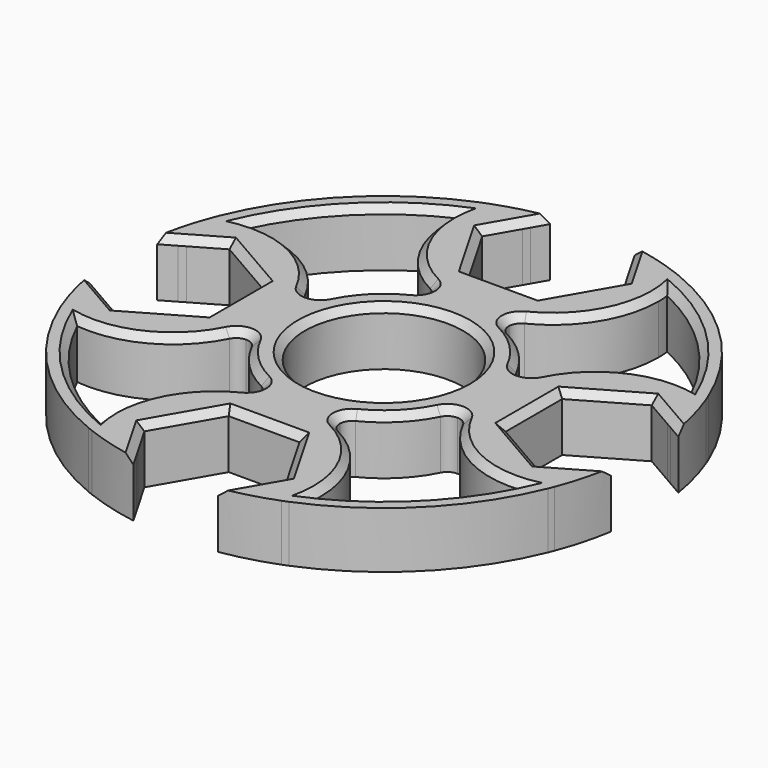
from build123d import *

# Parameters (mm, degrees)
F0_R          = 11.25
F1_DEPTH      = 8
F2_T6_DEPTH   = 13.2460185776
F2_T10_DEPTH  = 15.1933659759
F2_T15_DEPTH  = 15.1933659759
F2_T20_DEPTH  = 15.1933659759
F2_T25_DEPTH  = 13.2460185776
F2_T29_DEPTH  = 15.1933659759
F2_T34_DEPTH  = 13.2460185776
F2_T38_DEPTH  = 15.1933659759
F2_T43_DEPTH  = 15.1933659759
F2_T48_DEPTH  = 13.2460185776
F2_T52_ANGLE  = 79.6397986482
F2_S53_R      = 35
F2_T54_DEPTH  = 11
F2_T57_ANGLE  = 79.6397986482
F2_S58_R      = 35
F2_T59_DEPTH  = 11
F2_T62_ANGLE  = 48.0029281472
F2_S63_R      = 15
F2_T64_DEPTH  = 16
F2_S65_R      = 15
F2_T66_DEPTH  = 16
F2_T69_ANGLE  = 48.0029281472
F2_S70_R      = 15
F2_T71_DEPTH  = 16
F2_S72_R      = 15
F2_T73_DEPTH  = 16
F2_T76_DEPTH  = 13.2460185776
F2_T80_DEPTH  = 15.1933659759
F2_T85_DEPTH  = 15.1933659759
F2_T90_DEPTH  = 15.1933659759
F2_T95_DEPTH  = 13.2460185776
F2_T99_ANGLE  = 79.6397986482
F2_S100_R     = 35
F2_T101_DEPTH = 11
F2_T104_ANGLE = 48.0029281472
F2_S105_R     = 15
F2_T106_DEPTH = 16
F2_S107_R     = 15
F2_T108_DEPTH = 16
F2_T111_DEPTH = 13.2460185776
F2_T115_DEPTH = 15.1933659759
F2_T120_DEPTH = 15.1933659759
F2_T125_DEPTH = 15.1933659759
F2_T130_DEPTH = 13.2460185776
F2_T134_ANGLE = 79.6397986482
F2_S135_R     = 35
F2_T136_DEPTH = 11
F2_T139_ANGLE = 48.0029281472
F2_S140_R     = 15
F2_T141_DEPTH = 16
F2_S142_R     = 15
F2_T143_DEPTH = 16
F2_T146_ANGLE = 79.6397986482
F2_S147_R     = 35
F2_T148_DEPTH = 11
F2_T151_ANGLE = 126.8698976458
F2_T154_ANGLE = 36.8698976458
F2_T157_ANGLE = 126.8698976458
F2_T160_ANGLE = 126.8698976458
F2_T163_ANGLE = 36.8698976458
F2_T166_ANGLE = 126.8698976458
F2_T169_ANGLE = 79.6397986482
F2_S170_R     = 35
F2_T171_DEPTH = 11
F2_T174_ANGLE = 36.8698976458
F2_T177_ANGLE = 126.8698976458
F2_T180_ANGLE = 79.6397986482
F2_S181_R     = 35
F2_T182_DEPTH = 11
F2_T185_ANGLE = 126.8698976458
F2_T188_ANGLE = 36.8698976458
F2_T191_ANGLE = 126.8698976458
F2_T194_ANGLE = 79.6397986482
F2_S195_R     = 35
F2_T196_DEPTH = 11
F2_T199_ANGLE = 126.8698976458
F2_T203_DEPTH = 15.1933659759
F2_T207_DEPTH = 13.2460185776
F2_T213_DEPTH = 15.1933659759
F2_T217_DEPTH = 15.1933659759
F2_T223_DEPTH = 15.1933659759
F2_T227_DEPTH = 15.1933659759
F2_T233_DEPTH = 13.2460185776
F2_T237_DEPTH = 15.1933659759
F2_T243_DEPTH = 15.1933659759
F2_T247_DEPTH = 15.1933659759
F2_T253_DEPTH = 15.1933659759
F2_T257_DEPTH = 13.2460185776
F2_T263_DEPTH = 15.1933659759
F2_T267_DEPTH = 15.1933659759
F2_T273_DEPTH = 13.2460185776
F2_T277_DEPTH = 15.1933659759
F2_T283_ANGLE = 79.6397986482
F2_S284_R     = 35
F2_T285_DEPTH = 11
F2_T288_ANGLE = 48.0029281472
F2_S289_R     = 15
F2_T290_DEPTH = 16
F2_T295_ANGLE = 79.6397986482
F2_S296_R     = 35
F2_T297_DEPTH = 11
F2_T300_ANGLE = 48.0029281472
F2_S301_R     = 15
F2_T302_DEPTH = 16
F2_T307_ANGLE = 48.0029281472
F2_S308_R     = 15
F2_T309_DEPTH = 16
F2_T312_ANGLE = 79.6397986482
F2_S313_R     = 35
F2_T314_DEPTH = 11
F2_T319_ANGLE = 48.0029281472
F2_S320_R     = 15
F2_T321_DEPTH = 16
F2_T324_ANGLE = 79.6397986482
F2_S325_R     = 35
F2_T326_DEPTH = 11
F2_T331_DEPTH = 15.1933659759
F2_T335_DEPTH = 13.2460185776
F2_T341_DEPTH = 15.1933659759
F2_T345_DEPTH = 15.1933659759
F2_T351_DEPTH = 15.1933659759
F2_T355_DEPTH = 15.1933659759
F2_T361_DEPTH = 13.2460185776
F2_T365_DEPTH = 15.1933659759
F2_T371_ANGLE = 79.6397986482
F2_S372_R     = 35
F2_T373_DEPTH = 11
F2_T376_ANGLE = 48.0029281472
F2_S377_R     = 15
F2_T378_DEPTH = 16
F2_T383_ANGLE = 79.6397986482
F2_S384_R     = 35
F2_T385_DEPTH = 11
F2_T388_ANGLE = 48.0029281472
F2_S389_R     = 15
F2_T390_DEPTH = 16
F2_T395_DEPTH = 15.1933659759
F2_T399_DEPTH = 13.2460185776
F2_T405_DEPTH = 15.1933659759
F2_T409_DEPTH = 15.1933659759
F2_T415_DEPTH = 15.1933659759
F2_T419_DEPTH = 15.1933659759
F2_T425_DEPTH = 15.1933659759
F2_T429_DEPTH = 13.2460185776
F2_T435_ANGLE = 79.6397986482
F2_S436_R     = 35
F2_T437_DEPTH = 11
F2_T440_ANGLE = 48.0029281472
F2_S441_R     = 15
F2_T442_DEPTH = 16
F2_T447_ANGLE = 48.0029281472
F2_S448_R     = 15
F2_T449_DEPTH = 16
F2_T452_ANGLE = 79.6397986482
F2_S453_R     = 35
F2_T454_DEPTH = 11


# Not quite as in the source:
# - a fillet or chamfer that OpenCascade refuses, or shapes differently, is made with other operations: its cross-section is extruded or revolved along the edge and cut away or added


with BuildPart() as f1:
    # F0 (on Top) → F1 (new body)
    with BuildSketch(Plane.XY):
        with BuildLine():
            ThreePointArc((-16.583592135, 6.7082039325), (-22.8362258472, 13.1787837029), (-31.6666666667, 14.90711985))
            ThreePointArc((-31.6666666667, 14.90711985), (-33.1092804377, 11.3479314811), (-34.1532596523, 7.6521144217))
            Line((-34.1532596523, 7.6521144217), (-30, 10.05))
            Line((-30, 10.05), (-21.296444692, 5.025))
            Line((-21.296444692, 5.025), (-21.296444692, 0))
            Line((-21.296444692, 0), (-15, 0))
            ThreePointArc((-15, 0), (-15.401265158, 3.4462938082), (-16.583592135, 6.7082039325))
        make_face()
        with BuildLine():
            ThreePointArc((-34.1532596523, -7.6521144217), (-33.1092804377, -11.3479314811), (-31.6666666667, -14.90711985))
            ThreePointArc((-31.6666666667, -14.90711985), (-22.8362258472, -13.1787837029), (-16.583592135, -6.7082039325))
            ThreePointArc((-16.583592135, -6.7082039325), (-15.401265158, -3.4462938082), (-15, 0))
            Line((-15, 0), (-21.296444692, 0))
            Line((-21.296444692, 0), (-21.296444692, -5.025))
            Line((-21.296444692, -5.025), (-30, -10.05))
            Line((-30, -10.05), (-34.1532596523, -7.6521144217))
        make_face()
        with BuildLine():
            ThreePointArc((-34.6875, -14.248766394), (-33.1940907666, -14.6559811741), (-31.6666666667, -14.90711985))
            ThreePointArc((-31.6666666667, -14.90711985), (-33.1092804377, -11.3479314811), (-34.1532596523, -7.6521144217))
            Line((-34.1532596523, -7.6521144217), (-35, -7.1632486541))
            Line((-35, -7.1632486541), (-35, -13.4629120178))
            ThreePointArc((-35, -13.4629120178), (-34.8459654169, -13.8567201806), (-34.6875, -14.248766394))
        make_face()
        with BuildLine():
            ThreePointArc((-37.0171029911, -5.9986736992), (-36.2014432616, -9.7829190825), (-35, -13.4629120178))
            Line((-35, -13.4629120178), (-35, -7.1632486541))
            Line((-35, -7.1632486541), (-37.0171029911, -5.9986736992))
        make_face()
        with BuildLine():
            Line((-35, 7.1632486541), (-35, 13.4629120178))
            ThreePointArc((-35, 13.4629120178), (-36.2014432616, 9.7829190825), (-37.0171029911, 5.9986736992))
            Line((-37.0171029911, 5.9986736992), (-35, 7.1632486541))
        make_face()
        with BuildLine():
            ThreePointArc((-34.1532596523, 7.6521144217), (-33.1092804377, 11.3479314811), (-31.6666666667, 14.90711985))
            ThreePointArc((-31.6666666667, 14.90711985), (-33.1940907666, 14.6559811741), (-34.6875, 14.248766394))
            ThreePointArc((-34.6875, 14.248766394), (-34.8459654169, 13.8567201806), (-35, 13.4629120178))
            Line((-35, 13.4629120178), (-35, 7.1632486541))
            Line((-35, 7.1632486541), (-34.1532596523, 7.6521144217))
        make_face()
        with BuildLine():
            ThreePointArc((-31.6666666667, 14.90711985), (-24.7487373415, 24.7487373415), (-14.90711985, 31.6666666667))
            ThreePointArc((-14.90711985, 31.6666666667), (-14.6559811741, 33.1940907666), (-14.248766394, 34.6875))
            ThreePointArc((-14.248766394, 34.6875), (-26.5165042945, 26.5165042945), (-34.6875, 14.248766394))
            ThreePointArc((-34.6875, 14.248766394), (-33.1940907666, 14.6559811741), (-31.6666666667, 14.90711985))
        make_face()
        with BuildLine():
            ThreePointArc((-14.248766394, -34.6875), (-14.6559811741, -33.1940907666), (-14.90711985, -31.6666666667))
            ThreePointArc((-14.90711985, -31.6666666667), (-24.7487373415, -24.7487373415), (-31.6666666667, -14.90711985))
            ThreePointArc((-31.6666666667, -14.90711985), (-33.1940907666, -14.6559811741), (-34.6875, -14.248766394))
            ThreePointArc((-34.6875, -14.248766394), (-26.5165042945, -26.5165042945), (-14.248766394, -34.6875))
        make_face()
        with BuildLine():
            Line((-15, -5.7294901688), (-15, 0))
            ThreePointArc((-15, 0), (-15.401265158, -3.4462938082), (-16.583592135, -6.7082039325))
            ThreePointArc((-16.583592135, -6.7082039325), (-15.9308121026, -5.9939143809), (-15, -5.7294901688))
        make_face()
        with BuildLine():
            ThreePointArc((-15, -5.7294901688), (-14.0691878974, -5.9939143809), (-13.416407865, -6.7082039325))
            ThreePointArc((-13.416407865, -6.7082039325), (-14.598734842, -3.4462938082), (-15, 0))
            Line((-15, 0), (-15, -5.7294901688))
        make_face()
        with BuildLine():
            ThreePointArc((-15, 5.7294901688), (-15.9308121026, 5.9939143809), (-16.583592135, 6.7082039325))
            ThreePointArc((-16.583592135, 6.7082039325), (-15.401265158, 3.4462938082), (-15, 0))
            Line((-15, 0), (-15, 5.7294901688))
        make_face()
        with BuildLine():
            ThreePointArc((-15, 0), (-14.598734842, 3.4462938082), (-13.416407865, 6.7082039325))
            ThreePointArc((-13.416407865, 6.7082039325), (-14.0691878974, 5.9939143809), (-15, 5.7294901688))
            Line((-15, 5.7294901688), (-15, 0))
        make_face()
        with BuildLine():
            ThreePointArc((-14.90711985, -31.6666666667), (-11.3479314811, -33.1092804377), (-7.6521144217, -34.1532596523))
            Line((-7.6521144217, -34.1532596523), (-10.05, -30))
            Line((-10.05, -30), (-5.025, -21.296444692))
            Line((-5.025, -21.296444692), (0, -21.296444692))
            Line((0, -21.296444692), (0, -15))
            ThreePointArc((0, -15), (-3.4462938082, -15.401265158), (-6.7082039325, -16.583592135))
            ThreePointArc((-6.7082039325, -16.583592135), (-13.1787837029, -22.8362258472), (-14.90711985, -31.6666666667))
        make_face()
        with BuildLine():
            Line((-7.1632486541, -35), (-7.6521144217, -34.1532596523))
            ThreePointArc((-7.6521144217, -34.1532596523), (-11.3479314811, -33.1092804377), (-14.90711985, -31.6666666667))
            ThreePointArc((-14.90711985, -31.6666666667), (-14.6559811741, -33.1940907666), (-14.248766394, -34.6875))
            ThreePointArc((-14.248766394, -34.6875), (-13.8567201806, -34.8459654169), (-13.4629120178, -35))
            Line((-13.4629120178, -35), (-7.1632486541, -35))
        make_face()
        with BuildLine():
            Line((-5.9986736992, -37.0171029911), (-7.1632486541, -35))
            Line((-7.1632486541, -35), (-13.4629120178, -35))
            ThreePointArc((-13.4629120178, -35), (-9.7829190825, -36.2014432616), (-5.9986736992, -37.0171029911))
        make_face()
        with BuildLine():
            Line((13.4629120178, -35), (7.1632486541, -35))
            Line((7.1632486541, -35), (5.9986736992, -37.0171029911))
            ThreePointArc((5.9986736992, -37.0171029911), (9.7829190825, -36.2014432616), (13.4629120178, -35))
        make_face()
        with BuildLine():
            ThreePointArc((14.248766394, -34.6875), (14.6559811741, -33.1940907666), (14.90711985, -31.6666666667))
            ThreePointArc((14.90711985, -31.6666666667), (11.3479314811, -33.1092804377), (7.6521144217, -34.1532596523))
            Line((7.6521144217, -34.1532596523), (7.1632486541, -35))
            Line((7.1632486541, -35), (13.4629120178, -35))
            ThreePointArc((13.4629120178, -35), (13.8567201806, -34.8459654169), (14.248766394, -34.6875))
        make_face()
        with BuildLine():
            ThreePointArc((7.6521144217, -34.1532596523), (11.3479314811, -33.1092804377), (14.90711985, -31.6666666667))
            ThreePointArc((14.90711985, -31.6666666667), (14.9767619623, -30.8346263386), (15, -30))
            ThreePointArc((15, -30), (12.7597621253, -22.1140333182), (6.7082039325, -16.583592135))
            ThreePointArc((6.7082039325, -16.583592135), (3.4462938082, -15.401265158), (0, -15))
            Line((0, -15), (0, -21.296444692))
            Line((0, -21.296444692), (5.025, -21.296444692))
            Line((5.025, -21.296444692), (10.05, -30))
            Line((10.05, -30), (7.6521144217, -34.1532596523))
        make_face()
        with BuildLine():
            ThreePointArc((34.6875, -14.248766394), (33.1940907666, -14.6559811741), (31.6666666667, -14.90711985))
            ThreePointArc((31.6666666667, -14.90711985), (24.7487373415, -24.7487373415), (14.90711985, -31.6666666667))
            ThreePointArc((14.90711985, -31.6666666667), (14.6559811741, -33.1940907666), (14.248766394, -34.6875))
            ThreePointArc((14.248766394, -34.6875), (26.5165042945, -26.5165042945), (34.6875, -14.248766394))
        make_face()
        with BuildLine():
            Line((35, -7.1632486541), (34.1532596523, -7.6521144217))
            ThreePointArc((34.1532596523, -7.6521144217), (33.1092804377, -11.3479314811), (31.6666666667, -14.90711985))
            ThreePointArc((31.6666666667, -14.90711985), (33.1940907666, -14.6559811741), (34.6875, -14.248766394))
            ThreePointArc((34.6875, -14.248766394), (34.8459654169, -13.8567201806), (35, -13.4629120178))
            Line((35, -13.4629120178), (35, -7.1632486541))
        make_face()
        with BuildLine():
            Line((37.0171029911, -5.9986736992), (35, -7.1632486541))
            Line((35, -7.1632486541), (35, -13.4629120178))
            ThreePointArc((35, -13.4629120178), (36.2014432616, -9.7829190825), (37.0171029911, -5.9986736992))
        make_face()
        with BuildLine():
            ThreePointArc((31.6666666667, -14.90711985), (33.1092804377, -11.3479314811), (34.1532596523, -7.6521144217))
            Line((34.1532596523, -7.6521144217), (30, -10.05))
            Line((30, -10.05), (21.296444692, -5.025))
            Line((21.296444692, -5.025), (21.296444692, 0))
            Line((21.296444692, 0), (15, 0))
            ThreePointArc((15, 0), (15.401265158, -3.4462938082), (16.583592135, -6.7082039325))
            ThreePointArc((16.583592135, -6.7082039325), (22.8362258472, -13.1787837029), (31.6666666667, -14.90711985))
        make_face()
        with BuildLine():
            Line((30, 10.05), (34.1532596523, 7.6521144217))
            ThreePointArc((34.1532596523, 7.6521144217), (33.1092804377, 11.3479314811), (31.6666666667, 14.90711985))
            ThreePointArc((31.6666666667, 14.90711985), (22.8362258472, 13.1787837029), (16.583592135, 6.7082039325))
            ThreePointArc((16.583592135, 6.7082039325), (15.401265158, 3.4462938082), (15, 0))
            Line((15, 0), (21.296444692, 0))
            Line((21.296444692, 0), (21.296444692, 5.025))
            Line((21.296444692, 5.025), (30, 10.05))
        make_face()
        with BuildLine():
            ThreePointArc((31.6666666667, 14.90711985), (33.1092804377, 11.3479314811), (34.1532596523, 7.6521144217))
            Line((34.1532596523, 7.6521144217), (35, 7.1632486541))
            Line((35, 7.1632486541), (35, 13.4629120178))
            ThreePointArc((35, 13.4629120178), (34.8459654169, 13.8567201806), (34.6875, 14.248766394))
            ThreePointArc((34.6875, 14.248766394), (33.1940907666, 14.6559811741), (31.6666666667, 14.90711985))
        make_face()
        with BuildLine():
            Line((35, 13.4629120178), (35, 7.1632486541))
            Line((35, 7.1632486541), (37.0171029911, 5.9986736992))
            ThreePointArc((37.0171029911, 5.9986736992), (36.2014432616, 9.7829190825), (35, 13.4629120178))
        make_face()
        with BuildLine():
            ThreePointArc((14.90711985, 31.6666666667), (24.7487373415, 24.7487373415), (31.6666666667, 14.90711985))
            ThreePointArc((31.6666666667, 14.90711985), (33.1940907666, 14.6559811741), (34.6875, 14.248766394))
            ThreePointArc((34.6875, 14.248766394), (26.5165042945, 26.5165042945), (14.248766394, 34.6875))
            ThreePointArc((14.248766394, 34.6875), (14.6559811741, 33.1940907666), (14.90711985, 31.6666666667))
        make_face()
        with BuildLine():
            ThreePointArc((7.6521144217, 34.1532596523), (11.3479314811, 33.1092804377), (14.90711985, 31.6666666667))
            ThreePointArc((14.90711985, 31.6666666667), (14.6559811741, 33.1940907666), (14.248766394, 34.6875))
            ThreePointArc((14.248766394, 34.6875), (13.8567201806, 34.8459654169), (13.4629120178, 35))
            Line((13.4629120178, 35), (7.1632486541, 35))
            Line((7.1632486541, 35), (7.6521144217, 34.1532596523))
        make_face()
        with BuildLine():
            Line((5.9986736992, 37.0171029911), (7.1632486541, 35))
            Line((7.1632486541, 35), (13.4629120178, 35))
            ThreePointArc((13.4629120178, 35), (9.7829190825, 36.2014432616), (5.9986736992, 37.0171029911))
        make_face()
        with BuildLine():
            ThreePointArc((15, 30), (14.9767619623, 30.8346263386), (14.90711985, 31.6666666667))
            ThreePointArc((14.90711985, 31.6666666667), (11.3479314811, 33.1092804377), (7.6521144217, 34.1532596523))
            Line((7.6521144217, 34.1532596523), (10.05, 30))
            Line((10.05, 30), (5.025, 21.296444692))
            Line((5.025, 21.296444692), (0, 21.296444692))
            Line((0, 21.296444692), (0, 15))
            ThreePointArc((0, 15), (3.4462938082, 15.401265158), (6.7082039325, 16.583592135))
            ThreePointArc((6.7082039325, 16.583592135), (12.7597621253, 22.1140333182), (15, 30))
        make_face()
        with BuildLine():
            Line((-10.05, 30), (-7.6521144217, 34.1532596523))
            ThreePointArc((-7.6521144217, 34.1532596523), (-11.3479314811, 33.1092804377), (-14.90711985, 31.6666666667))
            ThreePointArc((-14.90711985, 31.6666666667), (-13.1787837029, 22.8362258472), (-6.7082039325, 16.583592135))
            ThreePointArc((-6.7082039325, 16.583592135), (-3.4462938082, 15.401265158), (0, 15))
            Line((0, 15), (0, 21.296444692))
            Line((0, 21.296444692), (-5.025, 21.296444692))
            Line((-5.025, 21.296444692), (-10.05, 30))
        make_face()
        with BuildLine():
            ThreePointArc((-14.90711985, 31.6666666667), (-11.3479314811, 33.1092804377), (-7.6521144217, 34.1532596523))
            Line((-7.6521144217, 34.1532596523), (-7.1632486541, 35))
            Line((-7.1632486541, 35), (-13.4629120178, 35))
            ThreePointArc((-13.4629120178, 35), (-13.8567201806, 34.8459654169), (-14.248766394, 34.6875))
            ThreePointArc((-14.248766394, 34.6875), (-14.6559811741, 33.1940907666), (-14.90711985, 31.6666666667))
        make_face()
        with BuildLine():
            Line((-13.4629120178, 35), (-7.1632486541, 35))
            Line((-7.1632486541, 35), (-5.9986736992, 37.0171029911))
            ThreePointArc((-5.9986736992, 37.0171029911), (-9.7829190825, 36.2014432616), (-13.4629120178, 35))
        make_face()
        with BuildLine():
            ThreePointArc((-6.7082039325, 13.416407865), (-3.4462938082, 14.598734842), (0, 15))
            Line((0, 15), (-5.7294901688, 15))
            ThreePointArc((-5.7294901688, 15), (-5.9939143809, 14.0691878974), (-6.7082039325, 13.416407865))
        make_face()
        with BuildLine():
            Line((-5.7294901688, 15), (0, 15))
            ThreePointArc((0, 15), (-3.4462938082, 15.401265158), (-6.7082039325, 16.583592135))
            ThreePointArc((-6.7082039325, 16.583592135), (-5.9939143809, 15.9308121026), (-5.7294901688, 15))
        make_face()
        with BuildLine():
            ThreePointArc((5.7294901688, 15), (5.9939143809, 15.9308121026), (6.7082039325, 16.583592135))
            ThreePointArc((6.7082039325, 16.583592135), (3.4462938082, 15.401265158), (0, 15))
            Line((0, 15), (5.7294901688, 15))
        make_face()
        with BuildLine():
            ThreePointArc((0, 15), (3.4462938082, 14.598734842), (6.7082039325, 13.416407865))
            ThreePointArc((6.7082039325, 13.416407865), (5.9939143809, 14.0691878974), (5.7294901688, 15))
            Line((5.7294901688, 15), (0, 15))
        make_face()
        with BuildLine():
            ThreePointArc((15, 0), (15.401265158, 3.4462938082), (16.583592135, 6.7082039325))
            ThreePointArc((16.583592135, 6.7082039325), (15.9308121026, 5.9939143809), (15, 5.7294901688))
            Line((15, 5.7294901688), (15, 0))
        make_face()
        with BuildLine():
            ThreePointArc((13.416407865, 6.7082039325), (14.598734842, 3.4462938082), (15, 0))
            Line((15, 0), (15, 5.7294901688))
            ThreePointArc((15, 5.7294901688), (14.0691878974, 5.9939143809), (13.416407865, 6.7082039325))
        make_face()
        with BuildLine():
            Line((15, -5.7294901688), (15, 0))
            ThreePointArc((15, 0), (14.598734842, -3.4462938082), (13.416407865, -6.7082039325))
            ThreePointArc((13.416407865, -6.7082039325), (14.0691878974, -5.9939143809), (15, -5.7294901688))
        make_face()
        with BuildLine():
            ThreePointArc((5.7294901688, -15), (5.9939143809, -14.0691878974), (6.7082039325, -13.416407865))
            ThreePointArc((6.7082039325, -13.416407865), (3.4462938082, -14.598734842), (0, -15))
            Line((0, -15), (5.7294901688, -15))
        make_face()
        with BuildLine():
            ThreePointArc((0, -15), (3.4462938082, -15.401265158), (6.7082039325, -16.583592135))
            ThreePointArc((6.7082039325, -16.583592135), (5.9939143809, -15.9308121026), (5.7294901688, -15))
            Line((5.7294901688, -15), (0, -15))
        make_face()
        with BuildLine():
            ThreePointArc((15, -5.7294901688), (15.9308121026, -5.9939143809), (16.583592135, -6.7082039325))
            ThreePointArc((16.583592135, -6.7082039325), (15.401265158, -3.4462938082), (15, 0))
            Line((15, 0), (15, -5.7294901688))
        make_face()
        with BuildLine():
            ThreePointArc((13.416407865, -6.7082039325), (14.598734842, -3.4462938082), (15, 0))
            ThreePointArc((15, 0), (14.598734842, 3.4462938082), (13.416407865, 6.7082039325))
            ThreePointArc((13.416407865, 6.7082039325), (10.6066017178, 10.6066017178), (6.7082039325, 13.416407865))
            ThreePointArc((6.7082039325, 13.416407865), (3.4462938082, 14.598734842), (0, 15))
            ThreePointArc((0, 15), (-3.4462938082, 14.598734842), (-6.7082039325, 13.416407865))
            ThreePointArc((-6.7082039325, 13.416407865), (-10.6066017178, 10.6066017178), (-13.416407865, 6.7082039325))
            ThreePointArc((-13.416407865, 6.7082039325), (-14.598734842, 3.4462938082), (-15, 0))
            ThreePointArc((-15, 0), (-14.598734842, -3.4462938082), (-13.416407865, -6.7082039325))
            ThreePointArc((-13.416407865, -6.7082039325), (-10.6066017178, -10.6066017178), (-6.7082039325, -13.416407865))
            ThreePointArc((-6.7082039325, -13.416407865), (-3.4462938082, -14.598734842), (0, -15))
            ThreePointArc((0, -15), (3.4462938082, -14.598734842), (6.7082039325, -13.416407865))
            ThreePointArc((6.7082039325, -13.416407865), (10.6066017178, -10.6066017178), (13.416407865, -6.7082039325))
        make_face()
        Circle(F0_R, mode=Mode.SUBTRACT)
        with BuildLine():
            ThreePointArc((-6.7082039325, -16.583592135), (-3.4462938082, -15.401265158), (0, -15))
            Line((0, -15), (-5.7294901688, -15))
            ThreePointArc((-5.7294901688, -15), (-5.9939143809, -15.9308121026), (-6.7082039325, -16.583592135))
        make_face()
        with BuildLine():
            Line((-5.7294901688, -15), (0, -15))
            ThreePointArc((0, -15), (-3.4462938082, -14.598734842), (-6.7082039325, -13.416407865))
            ThreePointArc((-6.7082039325, -13.416407865), (-5.9939143809, -14.0691878974), (-5.7294901688, -15))
        make_face()
    extrude(amount=F1_DEPTH)

    # F2: chamfer of 1 on 45 edges, made by hand


with BuildPart() as f2_tool1:
    # F2_s2 → F2_t3 (revolve)
    with BuildSketch(Plane.XZ):
        Polygon((11.25, 7), (12.25, 8), (11.25, 8), align=None)
    revolve(axis=Axis((0, 0, 8), (0, 0, 1)))


with BuildPart() as f2_tool4:
    # F2_s5 → F2_t6 (new body)
    with BuildSketch(Plane(origin=(9.1920395628, 15.9210795479, 0), x_dir=(0, 0, 1), z_dir=(0.5, 0.8660254038, 0))):
        Polygon((7, -23.703555308), (8, -24.703555308), (8, -23.703555308), align=None)
    extrude(amount=F2_T6_DEPTH)

    split(bisect_by=Plane(origin=(5.4528810568, 3.148222346, 0), x_dir=(0, 0, 1), z_dir=(0.8660254038, 0.5, 0)), keep=Keep.TOP)


with BuildPart() as f2_tool8:
    # F2_s9 → F2_t10 (new body)
    with BuildSketch(Plane(origin=(-9.1920395628, 15.9210795479, 0), x_dir=(0, 0, 1), z_dir=(-0.5, 0.8660254038, 0))):
        Polygon((7, 6.296444692), (8, 5.296444692), (8, 6.296444692), align=None)
    extrude(amount=F2_T10_DEPTH)

    split(bisect_by=Plane.XZ.offset(-21.296444692), keep=Keep.BOTTOM)

    split(bisect_by=Plane(origin=(-20.5278810568, 11.851777654, 0), x_dir=(0, 0, 1), z_dir=(0.8660254038, -0.5, 0)), keep=Keep.TOP)


with BuildPart() as f2_tool13:
    # F2_s14 → F2_t15 (new body)
    with BuildSketch(Plane.YZ.offset(7.596682988)):
        Polygon((21.296444692, 7), (20.296444692, 8), (21.296444692, 8), align=None)
    extrude(amount=-F2_T15_DEPTH)

    split(bisect_by=Plane(origin=(-5.4528810568, 3.148222346, 0), x_dir=(0, 0, 1), z_dir=(-0.8660254038, 0.5, 0)), keep=Keep.TOP)

    split(bisect_by=Plane(origin=(5.4528810568, 3.148222346, 0), x_dir=(0, 0, 1), z_dir=(0.8660254038, 0.5, 0)), keep=Keep.TOP)


with BuildPart() as f2_tool18:
    # F2_s19 → F2_t20 (new body)
    with BuildSketch(Plane(origin=(16.7887225507, 29.0789204521, 0), x_dir=(0, 0, 1), z_dir=(-0.5, -0.8660254038, 0))):
        Polygon((7, 6.296444692), (8, 5.296444692), (8, 6.296444692), align=None)
    extrude(amount=F2_T20_DEPTH)

    split(bisect_by=Plane(origin=(20.5278810568, 11.851777654, 0), x_dir=(0, 0, 1), z_dir=(-0.8660254038, -0.5, 0)), keep=Keep.TOP)

    split(bisect_by=Plane.XZ.offset(-21.296444692), keep=Keep.BOTTOM)


with BuildPart() as f2_tool23:
    # F2_s24 → F2_t25 (new body)
    with BuildSketch(Plane(origin=(-15.8150488516, 27.3924681351, 0), x_dir=(0, 0, 1), z_dir=(0.5, -0.8660254038, 0))):
        Polygon((7, -23.703555308), (8, -24.703555308), (8, -23.703555308), align=None)
    extrude(amount=F2_T25_DEPTH)

    split(bisect_by=Plane(origin=(-5.4528810568, 3.148222346, 0), x_dir=(0, 0, 1), z_dir=(-0.8660254038, 0.5, 0)), keep=Keep.TOP)


with BuildPart() as f2_tool27:
    # F2_s28 → F2_t29 (new body)
    with BuildSketch(Plane(origin=(15.9210795479, 9.1920395628, 0), x_dir=(0, 0, 1), z_dir=(0.8660254038, 0.5, 0))):
        Polygon((7, 6.296444692), (8, 5.296444692), (8, 6.296444692), align=None)
    extrude(amount=F2_T29_DEPTH)

    split(bisect_by=Plane.YZ.offset(21.296444692), keep=Keep.TOP)

    split(bisect_by=Plane(origin=(11.851777654, 20.5278810568, 0), x_dir=(0, 0, 1), z_dir=(-0.5, -0.8660254038, 0)), keep=Keep.TOP)


with BuildPart() as f2_tool32:
    # F2_s33 → F2_t34 (new body)
    with BuildSketch(Plane(origin=(15.9210795479, -9.1920395628, 0), x_dir=(0, 0, 1), z_dir=(0.8660254038, -0.5, 0))):
        Polygon((7, -23.703555308), (8, -24.703555308), (8, -23.703555308), align=None)
    extrude(amount=F2_T34_DEPTH)

    split(bisect_by=Plane(origin=(3.148222346, -5.4528810568, 0), x_dir=(0, 0, 1), z_dir=(0.5, -0.8660254038, 0)), keep=Keep.TOP)


with BuildPart() as f2_tool36:
    # F2_s37 → F2_t38 (new body)
    with BuildSketch(Plane.XZ.offset(7.596682988)):
        Polygon((21.296444692, 7), (20.296444692, 8), (21.296444692, 8), align=None)
    extrude(amount=-F2_T38_DEPTH)

    split(bisect_by=Plane(origin=(3.148222346, 5.4528810568, 0), x_dir=(0, 0, 1), z_dir=(0.5, 0.8660254038, 0)), keep=Keep.TOP)

    split(bisect_by=Plane(origin=(3.148222346, -5.4528810568, 0), x_dir=(0, 0, 1), z_dir=(0.5, -0.8660254038, 0)), keep=Keep.TOP)


with BuildPart() as f2_tool41:
    # F2_s42 → F2_t43 (new body)
    with BuildSketch(Plane(origin=(29.0789204521, -16.7887225507, 0), x_dir=(0, 0, 1), z_dir=(-0.8660254038, 0.5, 0))):
        Polygon((7, 6.296444692), (8, 5.296444692), (8, 6.296444692), align=None)
    extrude(amount=F2_T43_DEPTH)

    split(bisect_by=Plane(origin=(11.851777654, -20.5278810568, 0), x_dir=(0, 0, 1), z_dir=(-0.5, 0.8660254038, 0)), keep=Keep.TOP)

    split(bisect_by=Plane.YZ.offset(21.296444692), keep=Keep.TOP)


with BuildPart() as f2_tool46:
    # F2_s47 → F2_t48 (new body)
    with BuildSketch(Plane(origin=(27.3924681351, 15.8150488516, 0), x_dir=(0, 0, 1), z_dir=(-0.8660254038, -0.5, 0))):
        Polygon((7, -23.703555308), (8, -24.703555308), (8, -23.703555308), align=None)
    extrude(amount=F2_T48_DEPTH)

    split(bisect_by=Plane(origin=(3.148222346, 5.4528810568, 0), x_dir=(0, 0, 1), z_dir=(0.5, 0.8660254038, 0)), keep=Keep.TOP)


with BuildPart() as f2_tool50:
    # F2_s51 → F2_t52 (revolve)
    with BuildSketch(Plane(origin=(6, -12, 0), x_dir=(0, 0, 1), z_dir=(-0.4472135955, 0.894427191, 0))):
        Polygon((7, 11.83281573), (8, 12.83281573), (8, 11.83281573), align=None)
    revolve(axis=Axis((30, 0, 8), (0, 0, 1)), revolution_arc=F2_T52_ANGLE)

    # F2_s53 → F2_t54 (intersect, symmetric)
    with BuildSketch(Plane.XY.offset(7.5)):
        Circle(F2_S53_R)
    extrude(amount=F2_T54_DEPTH, both=True, mode=Mode.INTERSECT)


with BuildPart() as f2_tool55:
    # F2_s56 → F2_t57 (revolve)
    with BuildSketch(Plane(origin=(12, 6, 0), x_dir=(0, 0, 1), z_dir=(-0.894427191, -0.4472135955, 0))):
        Polygon((7, 11.83281573), (8, 12.83281573), (8, 11.83281573), align=None)
    revolve(axis=Axis((0, 30, 8), (0, 0, 1)), revolution_arc=F2_T57_ANGLE)

    # F2_s58 → F2_t59 (intersect, symmetric)
    with BuildSketch(Plane.XY.offset(7.5)):
        Circle(F2_S58_R)
    extrude(amount=F2_T59_DEPTH, both=True, mode=Mode.INTERSECT)


with BuildPart() as f2_tool60:
    # F2_s61 → F2_t62 (revolve)
    with BuildSketch(Plane(origin=(0, 0, 0), x_dir=(0, 0, 1), z_dir=(0.3583440937, 0.9335895835, 0))):
        Polygon((7, 35), (8, 36), (8, 35), align=None)
    revolve(axis=Axis((0, 0, 8), (0, 0, -1)), revolution_arc=F2_T62_ANGLE)

    # F2_s63 → F2_t64 (cut, symmetric)
    with BuildSketch(Plane.XY.offset(7.5)):
        with Locations((30, 0)):
            Circle(F2_S63_R)
    extrude(amount=F2_T64_DEPTH, both=True, mode=Mode.SUBTRACT)

    # F2_s65 → F2_t66 (cut, symmetric)
    with BuildSketch(Plane.XY.offset(7.5)):
        with Locations((0, -30)):
            Circle(F2_S65_R)
    extrude(amount=F2_T66_DEPTH, both=True, mode=Mode.SUBTRACT)


with BuildPart() as f2_tool67:
    # F2_s68 → F2_t69 (revolve)
    with BuildSketch(Plane(origin=(0, 0, 0), x_dir=(0, 0, 1), z_dir=(-0.9335895835, 0.3583440937, 0))):
        Polygon((7, 35), (8, 36), (8, 35), align=None)
    revolve(axis=Axis((0, 0, 8), (0, 0, -1)), revolution_arc=F2_T69_ANGLE)

    # F2_s70 → F2_t71 (cut, symmetric)
    with BuildSketch(Plane.XY.offset(7.5)):
        with Locations((0, 30)):
            Circle(F2_S70_R)
    extrude(amount=F2_T71_DEPTH, both=True, mode=Mode.SUBTRACT)

    # F2_s72 → F2_t73 (cut, symmetric)
    with BuildSketch(Plane.XY.offset(7.5)):
        with Locations((30, 0)):
            Circle(F2_S72_R)
    extrude(amount=F2_T73_DEPTH, both=True, mode=Mode.SUBTRACT)


with BuildPart() as f2_tool74:
    # F2_s75 → F2_t76 (new body)
    with BuildSketch(Plane(origin=(-9.1920395628, -15.9210795479, 0), x_dir=(0, 0, 1), z_dir=(-0.5, -0.8660254038, 0))):
        Polygon((7, -23.703555308), (8, -24.703555308), (8, -23.703555308), align=None)
    extrude(amount=F2_T76_DEPTH)

    split(bisect_by=Plane(origin=(-5.4528810568, -3.148222346, 0), x_dir=(0, 0, 1), z_dir=(-0.8660254038, -0.5, 0)), keep=Keep.TOP)


with BuildPart() as f2_tool78:
    # F2_s79 → F2_t80 (new body)
    with BuildSketch(Plane(origin=(9.1920395628, -15.9210795479, 0), x_dir=(0, 0, 1), z_dir=(0.5, -0.8660254038, 0))):
        Polygon((7, 6.296444692), (8, 5.296444692), (8, 6.296444692), align=None)
    extrude(amount=F2_T80_DEPTH)

    split(bisect_by=Plane.XZ.offset(21.296444692), keep=Keep.TOP)

    split(bisect_by=Plane(origin=(20.5278810568, -11.851777654, 0), x_dir=(0, 0, 1), z_dir=(-0.8660254038, 0.5, 0)), keep=Keep.TOP)


with BuildPart() as f2_tool83:
    # F2_s84 → F2_t85 (new body)
    with BuildSketch(Plane.YZ.offset(-7.596682988)):
        Polygon((-21.296444692, 7), (-20.296444692, 8), (-21.296444692, 8), align=None)
    extrude(amount=F2_T85_DEPTH)

    split(bisect_by=Plane(origin=(5.4528810568, -3.148222346, 0), x_dir=(0, 0, 1), z_dir=(0.8660254038, -0.5, 0)), keep=Keep.TOP)

    split(bisect_by=Plane(origin=(-5.4528810568, -3.148222346, 0), x_dir=(0, 0, 1), z_dir=(-0.8660254038, -0.5, 0)), keep=Keep.TOP)


with BuildPart() as f2_tool88:
    # F2_s89 → F2_t90 (new body)
    with BuildSketch(Plane(origin=(-16.7887225507, -29.0789204521, 0), x_dir=(0, 0, 1), z_dir=(0.5, 0.8660254038, 0))):
        Polygon((7, 6.296444692), (8, 5.296444692), (8, 6.296444692), align=None)
    extrude(amount=F2_T90_DEPTH)

    split(bisect_by=Plane(origin=(-20.5278810568, -11.851777654, 0), x_dir=(0, 0, 1), z_dir=(0.8660254038, 0.5, 0)), keep=Keep.TOP)

    split(bisect_by=Plane.XZ.offset(21.296444692), keep=Keep.TOP)


with BuildPart() as f2_tool93:
    # F2_s94 → F2_t95 (new body)
    with BuildSketch(Plane(origin=(15.8150488516, -27.3924681351, 0), x_dir=(0, 0, 1), z_dir=(-0.5, 0.8660254038, 0))):
        Polygon((7, -23.703555308), (8, -24.703555308), (8, -23.703555308), align=None)
    extrude(amount=F2_T95_DEPTH)

    split(bisect_by=Plane(origin=(5.4528810568, -3.148222346, 0), x_dir=(0, 0, 1), z_dir=(0.8660254038, -0.5, 0)), keep=Keep.TOP)


with BuildPart() as f2_tool97:
    # F2_s98 → F2_t99 (revolve)
    with BuildSketch(Plane(origin=(-27.6635580425, 8.0395458642, 0), x_dir=(0, 0, 1), z_dir=(-0.9602700669, 0.2790723895, 0))):
        Polygon((7, -23.372171685), (8, -22.372171685), (8, -23.372171685), align=None)
    revolve(axis=Axis((-30, 0, 8), (0, 0, 1)), revolution_arc=F2_T99_ANGLE)

    # F2_s100 → F2_t101 (intersect, symmetric)
    with BuildSketch(Plane.XY.offset(7.5)):
        Circle(F2_S100_R)
    extrude(amount=F2_T101_DEPTH, both=True, mode=Mode.INTERSECT)


with BuildPart() as f2_tool102:
    # F2_s103 → F2_t104 (revolve)
    with BuildSketch(Plane(origin=(0, 0, 0), x_dir=(0, 0, 1), z_dir=(0.9335895835, -0.3583440937, 0))):
        Polygon((7, 35), (8, 36), (8, 35), align=None)
    revolve(axis=Axis((0, 0, 8), (0, 0, -1)), revolution_arc=F2_T104_ANGLE)

    # F2_s105 → F2_t106 (cut, symmetric)
    with BuildSketch(Plane.XY.offset(7.5)):
        with Locations((-30, 0)):
            Circle(F2_S105_R)
    extrude(amount=F2_T106_DEPTH, both=True, mode=Mode.SUBTRACT)

    # F2_s107 → F2_t108 (cut, symmetric)
    with BuildSketch(Plane.XY.offset(7.5)):
        with Locations((0, -30)):
            Circle(F2_S107_R)
    extrude(amount=F2_T108_DEPTH, both=True, mode=Mode.SUBTRACT)


with BuildPart() as f2_tool109:
    # F2_s110 → F2_t111 (new body)
    with BuildSketch(Plane(origin=(-15.9210795479, 9.1920395628, 0), x_dir=(0, 0, 1), z_dir=(-0.8660254038, 0.5, 0))):
        Polygon((7, -23.703555308), (8, -24.703555308), (8, -23.703555308), align=None)
    extrude(amount=F2_T111_DEPTH)

    split(bisect_by=Plane(origin=(-3.148222346, 5.4528810568, 0), x_dir=(0, 0, 1), z_dir=(-0.5, 0.8660254038, 0)), keep=Keep.TOP)


with BuildPart() as f2_tool113:
    # F2_s114 → F2_t115 (new body)
    with BuildSketch(Plane(origin=(-15.9210795479, -9.1920395628, 0), x_dir=(0, 0, 1), z_dir=(-0.8660254038, -0.5, 0))):
        Polygon((7, 6.296444692), (8, 5.296444692), (8, 6.296444692), align=None)
    extrude(amount=F2_T115_DEPTH)

    split(bisect_by=Plane.YZ.offset(-21.296444692), keep=Keep.BOTTOM)

    split(bisect_by=Plane(origin=(-11.851777654, -20.5278810568, 0), x_dir=(0, 0, 1), z_dir=(0.5, 0.8660254038, 0)), keep=Keep.TOP)


with BuildPart() as f2_tool118:
    # F2_s119 → F2_t120 (new body)
    with BuildSketch(Plane.XZ.offset(-7.596682988)):
        Polygon((-21.296444692, 7), (-20.296444692, 8), (-21.296444692, 8), align=None)
    extrude(amount=F2_T120_DEPTH)

    split(bisect_by=Plane(origin=(-3.148222346, -5.4528810568, 0), x_dir=(0, 0, 1), z_dir=(-0.5, -0.8660254038, 0)), keep=Keep.TOP)

    split(bisect_by=Plane(origin=(-3.148222346, 5.4528810568, 0), x_dir=(0, 0, 1), z_dir=(-0.5, 0.8660254038, 0)), keep=Keep.TOP)


with BuildPart() as f2_tool123:
    # F2_s124 → F2_t125 (new body)
    with BuildSketch(Plane(origin=(-29.0789204521, 16.7887225507, 0), x_dir=(0, 0, 1), z_dir=(0.8660254038, -0.5, 0))):
        Polygon((7, 6.296444692), (8, 5.296444692), (8, 6.296444692), align=None)
    extrude(amount=F2_T125_DEPTH)

    split(bisect_by=Plane.YZ.offset(-21.296444692), keep=Keep.BOTTOM)

    split(bisect_by=Plane(origin=(-11.851777654, 20.5278810568, 0), x_dir=(0, 0, 1), z_dir=(0.5, -0.8660254038, 0)), keep=Keep.TOP)


with BuildPart() as f2_tool128:
    # F2_s129 → F2_t130 (new body)
    with BuildSketch(Plane(origin=(-27.3924681351, -15.8150488516, 0), x_dir=(0, 0, 1), z_dir=(0.8660254038, 0.5, 0))):
        Polygon((7, -23.703555308), (8, -24.703555308), (8, -23.703555308), align=None)
    extrude(amount=F2_T130_DEPTH)

    split(bisect_by=Plane(origin=(-3.148222346, -5.4528810568, 0), x_dir=(0, 0, 1), z_dir=(-0.5, -0.8660254038, 0)), keep=Keep.TOP)


with BuildPart() as f2_tool132:
    # F2_s133 → F2_t134 (revolve)
    with BuildSketch(Plane(origin=(-6, 12, 0), x_dir=(0, 0, 1), z_dir=(0.4472135955, -0.894427191, 0))):
        Polygon((7, 11.83281573), (8, 12.83281573), (8, 11.83281573), align=None)
    revolve(axis=Axis((-30, 0, 8), (0, 0, 1)), revolution_arc=F2_T134_ANGLE)

    # F2_s135 → F2_t136 (intersect, symmetric)
    with BuildSketch(Plane.XY.offset(7.5)):
        Circle(F2_S135_R)
    extrude(amount=F2_T136_DEPTH, both=True, mode=Mode.INTERSECT)


with BuildPart() as f2_tool137:
    # F2_s138 → F2_t139 (revolve)
    with BuildSketch(Plane(origin=(0, 0, 0), x_dir=(0, 0, 1), z_dir=(-0.3583440937, -0.9335895835, 0))):
        Polygon((7, 35), (8, 36), (8, 35), align=None)
    revolve(axis=Axis((0, 0, 8), (0, 0, -1)), revolution_arc=F2_T139_ANGLE)

    # F2_s140 → F2_t141 (cut, symmetric)
    with BuildSketch(Plane.XY.offset(7.5)):
        with Locations((-30, 0)):
            Circle(F2_S140_R)
    extrude(amount=F2_T141_DEPTH, both=True, mode=Mode.SUBTRACT)

    # F2_s142 → F2_t143 (cut, symmetric)
    with BuildSketch(Plane.XY.offset(7.5)):
        with Locations((0, 30)):
            Circle(F2_S142_R)
    extrude(amount=F2_T143_DEPTH, both=True, mode=Mode.SUBTRACT)


with BuildPart() as f2_tool144:
    # F2_s145 → F2_t146 (revolve)
    with BuildSketch(Plane(origin=(8.0395458642, 27.6635580425, 0), x_dir=(0, 0, 1), z_dir=(0.2790723895, 0.9602700669, 0))):
        Polygon((7, -23.372171685), (8, -22.372171685), (8, -23.372171685), align=None)
    revolve(axis=Axis((0, 30, 8), (0, 0, 1)), revolution_arc=F2_T146_ANGLE)

    # F2_s147 → F2_t148 (intersect, symmetric)
    with BuildSketch(Plane.XY.offset(7.5)):
        Circle(F2_S147_R)
    extrude(amount=F2_T148_DEPTH, both=True, mode=Mode.INTERSECT)


with BuildPart() as f2_tool149:
    # F2_s150 → F2_t151 (revolve)
    with BuildSketch(Plane(origin=(-12, 6, 0), x_dir=(0, 0, 1), z_dir=(-0.894427191, 0.4472135955, 0))):
        Polygon((7, 11.83281573), (8, 12.83281573), (8, 11.83281573), align=None)
    revolve(axis=Axis((-7.5, 15, 8), (0, 0, -1)), revolution_arc=F2_T151_ANGLE)


with BuildPart() as f2_tool152:
    # F2_s153 → F2_t154 (revolve)
    with BuildSketch(Plane(origin=(0, 0, 0), x_dir=(0, 0, 1), z_dir=(0.894427191, 0.4472135955, 0))):
        Polygon((7, -15), (8, -14), (8, -15), align=None)
    revolve(axis=Axis((0, 0, 8), (0, 0, 1)), revolution_arc=F2_T154_ANGLE)


with BuildPart() as f2_tool155:
    # F2_s156 → F2_t157 (revolve)
    with BuildSketch(Plane(origin=(0, 0, 0), x_dir=(0, 0, 1), z_dir=(0.4472135955, 0.894427191, 0))):
        Polygon((7, -15), (8, -14), (8, -15), align=None)
    revolve(axis=Axis((-15, 7.5, 8), (0, 0, -1)), revolution_arc=F2_T157_ANGLE)


with BuildPart() as f2_tool158:
    # F2_s159 → F2_t160 (revolve)
    with BuildSketch(Plane(origin=(-6, -12, 0), x_dir=(0, 0, 1), z_dir=(-0.4472135955, -0.894427191, 0))):
        Polygon((7, 11.83281573), (8, 12.83281573), (8, 11.83281573), align=None)
    revolve(axis=Axis((-15, -7.5, 8), (0, 0, -1)), revolution_arc=F2_T160_ANGLE)


with BuildPart() as f2_tool161:
    # F2_s162 → F2_t163 (revolve)
    with BuildSketch(Plane(origin=(0, 0, 0), x_dir=(0, 0, 1), z_dir=(-0.4472135955, 0.894427191, 0))):
        Polygon((7, -15), (8, -14), (8, -15), align=None)
    revolve(axis=Axis((0, 0, 8), (0, 0, 1)), revolution_arc=F2_T163_ANGLE)


with BuildPart() as f2_tool164:
    # F2_s165 → F2_t166 (revolve)
    with BuildSketch(Plane(origin=(0, 0, 0), x_dir=(0, 0, 1), z_dir=(-0.894427191, 0.4472135955, 0))):
        Polygon((7, -15), (8, -14), (8, -15), align=None)
    revolve(axis=Axis((-7.5, -15, 8), (0, 0, -1)), revolution_arc=F2_T166_ANGLE)


with BuildPart() as f2_tool167:
    # F2_s168 → F2_t169 (revolve)
    with BuildSketch(Plane(origin=(-12, -6, 0), x_dir=(0, 0, 1), z_dir=(0.894427191, 0.4472135955, 0))):
        Polygon((7, 11.83281573), (8, 12.83281573), (8, 11.83281573), align=None)
    revolve(axis=Axis((0, -30, 8), (0, 0, 1)), revolution_arc=F2_T169_ANGLE)

    # F2_s170 → F2_t171 (intersect, symmetric)
    with BuildSketch(Plane.XY.offset(7.5)):
        Circle(F2_S170_R)
    extrude(amount=F2_T171_DEPTH, both=True, mode=Mode.INTERSECT)


with BuildPart() as f2_tool172:
    # F2_s173 → F2_t174 (revolve)
    with BuildSketch(Plane(origin=(0, 0, 0), x_dir=(0, 0, 1), z_dir=(-0.894427191, -0.4472135955, 0))):
        Polygon((7, -15), (8, -14), (8, -15), align=None)
    revolve(axis=Axis((0, 0, 8), (0, 0, 1)), revolution_arc=F2_T174_ANGLE)


with BuildPart() as f2_tool175:
    # F2_s176 → F2_t177 (revolve)
    with BuildSketch(Plane(origin=(0, 0, 0), x_dir=(0, 0, 1), z_dir=(-0.4472135955, -0.894427191, 0))):
        Polygon((7, -15), (8, -14), (8, -15), align=None)
    revolve(axis=Axis((15, -7.5, 8), (0, 0, -1)), revolution_arc=F2_T177_ANGLE)


with BuildPart() as f2_tool178:
    # F2_s179 → F2_t180 (revolve)
    with BuildSketch(Plane(origin=(-8.0395458642, -27.6635580425, 0), x_dir=(0, 0, 1), z_dir=(-0.2790723895, -0.9602700669, 0))):
        Polygon((7, -23.372171685), (8, -22.372171685), (8, -23.372171685), align=None)
    revolve(axis=Axis((0, -30, 8), (0, 0, 1)), revolution_arc=F2_T180_ANGLE)

    # F2_s181 → F2_t182 (intersect, symmetric)
    with BuildSketch(Plane.XY.offset(7.5)):
        Circle(F2_S181_R)
    extrude(amount=F2_T182_DEPTH, both=True, mode=Mode.INTERSECT)


with BuildPart() as f2_tool183:
    # F2_s184 → F2_t185 (revolve)
    with BuildSketch(Plane(origin=(12, -6, 0), x_dir=(0, 0, 1), z_dir=(0.894427191, -0.4472135955, 0))):
        Polygon((7, 11.83281573), (8, 12.83281573), (8, 11.83281573), align=None)
    revolve(axis=Axis((7.5, -15, 8), (0, 0, -1)), revolution_arc=F2_T185_ANGLE)


with BuildPart() as f2_tool186:
    # F2_s187 → F2_t188 (revolve)
    with BuildSketch(Plane(origin=(0, 0, 0), x_dir=(0, 0, 1), z_dir=(0.4472135955, -0.894427191, 0))):
        Polygon((7, -15), (8, -14), (8, -15), align=None)
    revolve(axis=Axis((0, 0, 8), (0, 0, 1)), revolution_arc=F2_T188_ANGLE)


with BuildPart() as f2_tool189:
    # F2_s190 → F2_t191 (revolve)
    with BuildSketch(Plane(origin=(0, 0, 0), x_dir=(0, 0, 1), z_dir=(0.894427191, -0.4472135955, 0))):
        Polygon((7, -15), (8, -14), (8, -15), align=None)
    revolve(axis=Axis((7.5, 15, 8), (0, 0, -1)), revolution_arc=F2_T191_ANGLE)


with BuildPart() as f2_tool192:
    # F2_s193 → F2_t194 (revolve)
    with BuildSketch(Plane(origin=(27.6635580425, -8.0395458642, 0), x_dir=(0, 0, 1), z_dir=(0.9602700669, -0.2790723895, 0))):
        Polygon((7, -23.372171685), (8, -22.372171685), (8, -23.372171685), align=None)
    revolve(axis=Axis((30, 0, 8), (0, 0, 1)), revolution_arc=F2_T194_ANGLE)

    # F2_s195 → F2_t196 (intersect, symmetric)
    with BuildSketch(Plane.XY.offset(7.5)):
        Circle(F2_S195_R)
    extrude(amount=F2_T196_DEPTH, both=True, mode=Mode.INTERSECT)


with BuildPart() as f2_tool197:
    # F2_s198 → F2_t199 (revolve)
    with BuildSketch(Plane(origin=(6, 12, 0), x_dir=(0, 0, 1), z_dir=(0.4472135955, 0.894427191, 0))):
        Polygon((7, 11.83281573), (8, 12.83281573), (8, 11.83281573), align=None)
    revolve(axis=Axis((15, 7.5, 8), (0, 0, -1)), revolution_arc=F2_T199_ANGLE)


with BuildPart() as f2_tool201:
    # F2_s202 → F2_t203 (new body)
    with BuildSketch(Plane(origin=(-9.1920395628, 15.9210795479, 0), x_dir=(0, 0, 1), z_dir=(-0.5, 0.8660254038, 0))):
        Polygon((7, 6.296444692), (8, 5.296444692), (8, 6.296444692), align=None)
    extrude(amount=F2_T203_DEPTH)

    split(bisect_by=Plane(origin=(-20.5278810568, 11.851777654, 0), x_dir=(0, 0, 1), z_dir=(-0.8660254038, 0.5, 0)), keep=Keep.TOP)


with BuildPart() as f2_tool205:
    # F2_s206 → F2_t207 (new body)
    with BuildSketch(Plane(origin=(9.1920395628, 15.9210795479, 0), x_dir=(0, 0, 1), z_dir=(0.5, 0.8660254038, 0))):
        Polygon((7, -23.703555308), (8, -24.703555308), (8, -23.703555308), align=None)
    extrude(amount=F2_T207_DEPTH)

    split(bisect_by=Plane(origin=(5.4528810568, 3.148222346, 0), x_dir=(0, 0, 1), z_dir=(-0.8660254038, -0.5, 0)), keep=Keep.TOP)


with BuildPart() as f2_tool201_1:
    add(f2_tool201.part)

    # F2_t209: intersect F2_tool205
    add(f2_tool205.part, mode=Mode.INTERSECT)


with BuildPart() as f2_tool211:
    # F2_s212 → F2_t213 (new body)
    with BuildSketch(Plane.YZ.offset(7.596682988)):
        Polygon((21.296444692, 7), (20.296444692, 8), (21.296444692, 8), align=None)
    extrude(amount=-F2_T213_DEPTH)

    split(bisect_by=Plane(origin=(5.4528810568, 3.148222346, 0), x_dir=(0, 0, 1), z_dir=(-0.8660254038, -0.5, 0)), keep=Keep.TOP)


with BuildPart() as f2_tool215:
    # F2_s216 → F2_t217 (new body)
    with BuildSketch(Plane(origin=(-9.1920395628, 15.9210795479, 0), x_dir=(0, 0, 1), z_dir=(-0.5, 0.8660254038, 0))):
        Polygon((7, 6.296444692), (8, 5.296444692), (8, 6.296444692), align=None)
    extrude(amount=F2_T217_DEPTH)

    split(bisect_by=Plane.XZ.offset(-21.296444692), keep=Keep.TOP)


with BuildPart() as f2_tool211_1:
    add(f2_tool211.part)

    # F2_t219: intersect F2_tool215
    add(f2_tool215.part, mode=Mode.INTERSECT)


with BuildPart() as f2_tool221:
    # F2_s222 → F2_t223 (new body)
    with BuildSketch(Plane(origin=(16.7887225507, 29.0789204521, 0), x_dir=(0, 0, 1), z_dir=(-0.5, -0.8660254038, 0))):
        Polygon((7, 6.296444692), (8, 5.296444692), (8, 6.296444692), align=None)
    extrude(amount=F2_T223_DEPTH)

    split(bisect_by=Plane.XZ.offset(-21.296444692), keep=Keep.TOP)


with BuildPart() as f2_tool225:
    # F2_s226 → F2_t227 (new body)
    with BuildSketch(Plane.YZ.offset(7.596682988)):
        Polygon((21.296444692, 7), (20.296444692, 8), (21.296444692, 8), align=None)
    extrude(amount=-F2_T227_DEPTH)

    split(bisect_by=Plane(origin=(-5.4528810568, 3.148222346, 0), x_dir=(0, 0, 1), z_dir=(0.8660254038, -0.5, 0)), keep=Keep.TOP)


with BuildPart() as f2_tool221_1:
    add(f2_tool221.part)

    # F2_t229: intersect F2_tool225
    add(f2_tool225.part, mode=Mode.INTERSECT)


with BuildPart() as f2_tool231:
    # F2_s232 → F2_t233 (new body)
    with BuildSketch(Plane(origin=(-15.8150488516, 27.3924681351, 0), x_dir=(0, 0, 1), z_dir=(0.5, -0.8660254038, 0))):
        Polygon((7, -23.703555308), (8, -24.703555308), (8, -23.703555308), align=None)
    extrude(amount=F2_T233_DEPTH)

    split(bisect_by=Plane(origin=(-5.4528810568, 3.148222346, 0), x_dir=(0, 0, 1), z_dir=(0.8660254038, -0.5, 0)), keep=Keep.TOP)


with BuildPart() as f2_tool235:
    # F2_s236 → F2_t237 (new body)
    with BuildSketch(Plane(origin=(16.7887225507, 29.0789204521, 0), x_dir=(0, 0, 1), z_dir=(-0.5, -0.8660254038, 0))):
        Polygon((7, 6.296444692), (8, 5.296444692), (8, 6.296444692), align=None)
    extrude(amount=F2_T237_DEPTH)

    split(bisect_by=Plane(origin=(20.5278810568, 11.851777654, 0), x_dir=(0, 0, 1), z_dir=(0.8660254038, 0.5, 0)), keep=Keep.TOP)


with BuildPart() as f2_tool231_1:
    add(f2_tool231.part)

    # F2_t239: intersect F2_tool235
    add(f2_tool235.part, mode=Mode.INTERSECT)


with BuildPart() as f2_tool241:
    # F2_s242 → F2_t243 (new body)
    with BuildSketch(Plane.XZ.offset(7.596682988)):
        Polygon((21.296444692, 7), (20.296444692, 8), (21.296444692, 8), align=None)
    extrude(amount=-F2_T243_DEPTH)

    split(bisect_by=Plane(origin=(3.148222346, -5.4528810568, 0), x_dir=(0, 0, 1), z_dir=(-0.5, 0.8660254038, 0)), keep=Keep.TOP)


with BuildPart() as f2_tool245:
    # F2_s246 → F2_t247 (new body)
    with BuildSketch(Plane(origin=(15.9210795479, 9.1920395628, 0), x_dir=(0, 0, 1), z_dir=(0.8660254038, 0.5, 0))):
        Polygon((7, 6.296444692), (8, 5.296444692), (8, 6.296444692), align=None)
    extrude(amount=F2_T247_DEPTH)

    split(bisect_by=Plane.YZ.offset(21.296444692), keep=Keep.BOTTOM)


with BuildPart() as f2_tool241_1:
    add(f2_tool241.part)

    # F2_t249: intersect F2_tool245
    add(f2_tool245.part, mode=Mode.INTERSECT)


with BuildPart() as f2_tool251:
    # F2_s252 → F2_t253 (new body)
    with BuildSketch(Plane(origin=(15.9210795479, 9.1920395628, 0), x_dir=(0, 0, 1), z_dir=(0.8660254038, 0.5, 0))):
        Polygon((7, 6.296444692), (8, 5.296444692), (8, 6.296444692), align=None)
    extrude(amount=F2_T253_DEPTH)

    split(bisect_by=Plane(origin=(11.851777654, 20.5278810568, 0), x_dir=(0, 0, 1), z_dir=(0.5, 0.8660254038, 0)), keep=Keep.TOP)


with BuildPart() as f2_tool255:
    # F2_s256 → F2_t257 (new body)
    with BuildSketch(Plane(origin=(15.9210795479, -9.1920395628, 0), x_dir=(0, 0, 1), z_dir=(0.8660254038, -0.5, 0))):
        Polygon((7, -23.703555308), (8, -24.703555308), (8, -23.703555308), align=None)
    extrude(amount=F2_T257_DEPTH)

    split(bisect_by=Plane(origin=(3.148222346, -5.4528810568, 0), x_dir=(0, 0, 1), z_dir=(-0.5, 0.8660254038, 0)), keep=Keep.TOP)


with BuildPart() as f2_tool251_1:
    add(f2_tool251.part)

    # F2_t259: intersect F2_tool255
    add(f2_tool255.part, mode=Mode.INTERSECT)


with BuildPart() as f2_tool261:
    # F2_s262 → F2_t263 (new body)
    with BuildSketch(Plane(origin=(29.0789204521, -16.7887225507, 0), x_dir=(0, 0, 1), z_dir=(-0.8660254038, 0.5, 0))):
        Polygon((7, 6.296444692), (8, 5.296444692), (8, 6.296444692), align=None)
    extrude(amount=F2_T263_DEPTH)

    split(bisect_by=Plane.YZ.offset(21.296444692), keep=Keep.BOTTOM)


with BuildPart() as f2_tool265:
    # F2_s266 → F2_t267 (new body)
    with BuildSketch(Plane.XZ.offset(7.596682988)):
        Polygon((21.296444692, 7), (20.296444692, 8), (21.296444692, 8), align=None)
    extrude(amount=-F2_T267_DEPTH)

    split(bisect_by=Plane(origin=(3.148222346, 5.4528810568, 0), x_dir=(0, 0, 1), z_dir=(-0.5, -0.8660254038, 0)), keep=Keep.TOP)


with BuildPart() as f2_tool261_1:
    add(f2_tool261.part)

    # F2_t269: intersect F2_tool265
    add(f2_tool265.part, mode=Mode.INTERSECT)


with BuildPart() as f2_tool271:
    # F2_s272 → F2_t273 (new body)
    with BuildSketch(Plane(origin=(27.3924681351, 15.8150488516, 0), x_dir=(0, 0, 1), z_dir=(-0.8660254038, -0.5, 0))):
        Polygon((7, -23.703555308), (8, -24.703555308), (8, -23.703555308), align=None)
    extrude(amount=F2_T273_DEPTH)

    split(bisect_by=Plane(origin=(3.148222346, 5.4528810568, 0), x_dir=(0, 0, 1), z_dir=(-0.5, -0.8660254038, 0)), keep=Keep.TOP)


with BuildPart() as f2_tool275:
    # F2_s276 → F2_t277 (new body)
    with BuildSketch(Plane(origin=(29.0789204521, -16.7887225507, 0), x_dir=(0, 0, 1), z_dir=(-0.8660254038, 0.5, 0))):
        Polygon((7, 6.296444692), (8, 5.296444692), (8, 6.296444692), align=None)
    extrude(amount=F2_T277_DEPTH)

    split(bisect_by=Plane(origin=(11.851777654, -20.5278810568, 0), x_dir=(0, 0, 1), z_dir=(0.5, -0.8660254038, 0)), keep=Keep.TOP)


with BuildPart() as f2_tool271_1:
    add(f2_tool271.part)

    # F2_t279: intersect F2_tool275
    add(f2_tool275.part, mode=Mode.INTERSECT)


with BuildPart() as f2_tool281:
    # F2_s282 → F2_t283 (revolve)
    with BuildSketch(Plane(origin=(6, -12, 0), x_dir=(0, 0, 1), z_dir=(-0.4472135955, 0.894427191, 0))):
        Polygon((7, 11.83281573), (8, 12.83281573), (8, 11.83281573), align=None)
    revolve(axis=Axis((30, 0, 8), (0, 0, 1)), revolution_arc=F2_T283_ANGLE)

    # F2_s284 → F2_t285 (cut, symmetric)
    with BuildSketch(Plane.XY.offset(7.5)):
        Circle(F2_S284_R)
    extrude(amount=F2_T285_DEPTH, both=True, mode=Mode.SUBTRACT)


with BuildPart() as f2_tool286:
    # F2_s287 → F2_t288 (revolve)
    with BuildSketch(Plane(origin=(0, 0, 0), x_dir=(0, 0, 1), z_dir=(0.3583440937, 0.9335895835, 0))):
        Polygon((7, 35), (8, 36), (8, 35), align=None)
    revolve(axis=Axis((0, 0, 8), (0, 0, -1)), revolution_arc=F2_T288_ANGLE)

    # F2_s289 → F2_t290 (intersect, symmetric)
    with BuildSketch(Plane.XY.offset(7.5)):
        with Locations((30, 0)):
            Circle(F2_S289_R)
    extrude(amount=F2_T290_DEPTH, both=True, mode=Mode.INTERSECT)


with BuildPart() as f2_tool281_1:
    add(f2_tool281.part)

    # F2_t291: intersect F2_tool286
    add(f2_tool286.part, mode=Mode.INTERSECT)


with BuildPart() as f2_tool293:
    # F2_s294 → F2_t295 (revolve)
    with BuildSketch(Plane(origin=(12, 6, 0), x_dir=(0, 0, 1), z_dir=(-0.894427191, -0.4472135955, 0))):
        Polygon((7, 11.83281573), (8, 12.83281573), (8, 11.83281573), align=None)
    revolve(axis=Axis((0, 30, 8), (0, 0, 1)), revolution_arc=F2_T295_ANGLE)

    # F2_s296 → F2_t297 (cut, symmetric)
    with BuildSketch(Plane.XY.offset(7.5)):
        Circle(F2_S296_R)
    extrude(amount=F2_T297_DEPTH, both=True, mode=Mode.SUBTRACT)


with BuildPart() as f2_tool298:
    # F2_s299 → F2_t300 (revolve)
    with BuildSketch(Plane(origin=(0, 0, 0), x_dir=(0, 0, 1), z_dir=(-0.9335895835, 0.3583440937, 0))):
        Polygon((7, 35), (8, 36), (8, 35), align=None)
    revolve(axis=Axis((0, 0, 8), (0, 0, -1)), revolution_arc=F2_T300_ANGLE)

    # F2_s301 → F2_t302 (intersect, symmetric)
    with BuildSketch(Plane.XY.offset(7.5)):
        with Locations((0, 30)):
            Circle(F2_S301_R)
    extrude(amount=F2_T302_DEPTH, both=True, mode=Mode.INTERSECT)


with BuildPart() as f2_tool293_1:
    add(f2_tool293.part)

    # F2_t303: intersect F2_tool298
    add(f2_tool298.part, mode=Mode.INTERSECT)


with BuildPart() as f2_tool305:
    # F2_s306 → F2_t307 (revolve)
    with BuildSketch(Plane(origin=(0, 0, 0), x_dir=(0, 0, 1), z_dir=(0.3583440937, 0.9335895835, 0))):
        Polygon((7, 35), (8, 36), (8, 35), align=None)
    revolve(axis=Axis((0, 0, 8), (0, 0, -1)), revolution_arc=F2_T307_ANGLE)

    # F2_s308 → F2_t309 (intersect, symmetric)
    with BuildSketch(Plane.XY.offset(7.5)):
        with Locations((0, -30)):
            Circle(F2_S308_R)
    extrude(amount=F2_T309_DEPTH, both=True, mode=Mode.INTERSECT)


with BuildPart() as f2_tool310:
    # F2_s311 → F2_t312 (revolve)
    with BuildSketch(Plane(origin=(-8.0395458642, -27.6635580425, 0), x_dir=(0, 0, 1), z_dir=(-0.2790723895, -0.9602700669, 0))):
        Polygon((7, -23.372171685), (8, -22.372171685), (8, -23.372171685), align=None)
    revolve(axis=Axis((0, -30, 8), (0, 0, 1)), revolution_arc=F2_T312_ANGLE)

    # F2_s313 → F2_t314 (cut, symmetric)
    with BuildSketch(Plane.XY.offset(7.5)):
        Circle(F2_S313_R)
    extrude(amount=F2_T314_DEPTH, both=True, mode=Mode.SUBTRACT)


with BuildPart() as f2_tool305_1:
    add(f2_tool305.part)

    # F2_t315: intersect F2_tool310
    add(f2_tool310.part, mode=Mode.INTERSECT)


with BuildPart() as f2_tool317:
    # F2_s318 → F2_t319 (revolve)
    with BuildSketch(Plane(origin=(0, 0, 0), x_dir=(0, 0, 1), z_dir=(-0.9335895835, 0.3583440937, 0))):
        Polygon((7, 35), (8, 36), (8, 35), align=None)
    revolve(axis=Axis((0, 0, 8), (0, 0, -1)), revolution_arc=F2_T319_ANGLE)

    # F2_s320 → F2_t321 (intersect, symmetric)
    with BuildSketch(Plane.XY.offset(7.5)):
        with Locations((30, 0)):
            Circle(F2_S320_R)
    extrude(amount=F2_T321_DEPTH, both=True, mode=Mode.INTERSECT)


with BuildPart() as f2_tool322:
    # F2_s323 → F2_t324 (revolve)
    with BuildSketch(Plane(origin=(27.6635580425, -8.0395458642, 0), x_dir=(0, 0, 1), z_dir=(0.9602700669, -0.2790723895, 0))):
        Polygon((7, -23.372171685), (8, -22.372171685), (8, -23.372171685), align=None)
    revolve(axis=Axis((30, 0, 8), (0, 0, 1)), revolution_arc=F2_T324_ANGLE)

    # F2_s325 → F2_t326 (cut, symmetric)
    with BuildSketch(Plane.XY.offset(7.5)):
        Circle(F2_S325_R)
    extrude(amount=F2_T326_DEPTH, both=True, mode=Mode.SUBTRACT)


with BuildPart() as f2_tool317_1:
    add(f2_tool317.part)

    # F2_t327: intersect F2_tool322
    add(f2_tool322.part, mode=Mode.INTERSECT)


with BuildPart() as f2_tool329:
    # F2_s330 → F2_t331 (new body)
    with BuildSketch(Plane(origin=(9.1920395628, -15.9210795479, 0), x_dir=(0, 0, 1), z_dir=(0.5, -0.8660254038, 0))):
        Polygon((7, 6.296444692), (8, 5.296444692), (8, 6.296444692), align=None)
    extrude(amount=F2_T331_DEPTH)

    split(bisect_by=Plane(origin=(20.5278810568, -11.851777654, 0), x_dir=(0, 0, 1), z_dir=(0.8660254038, -0.5, 0)), keep=Keep.TOP)


with BuildPart() as f2_tool333:
    # F2_s334 → F2_t335 (new body)
    with BuildSketch(Plane(origin=(-9.1920395628, -15.9210795479, 0), x_dir=(0, 0, 1), z_dir=(-0.5, -0.8660254038, 0))):
        Polygon((7, -23.703555308), (8, -24.703555308), (8, -23.703555308), align=None)
    extrude(amount=F2_T335_DEPTH)

    split(bisect_by=Plane(origin=(-5.4528810568, -3.148222346, 0), x_dir=(0, 0, 1), z_dir=(0.8660254038, 0.5, 0)), keep=Keep.TOP)


with BuildPart() as f2_tool329_1:
    add(f2_tool329.part)

    # F2_t337: intersect F2_tool333
    add(f2_tool333.part, mode=Mode.INTERSECT)


with BuildPart() as f2_tool339:
    # F2_s340 → F2_t341 (new body)
    with BuildSketch(Plane.YZ.offset(-7.596682988)):
        Polygon((-21.296444692, 7), (-20.296444692, 8), (-21.296444692, 8), align=None)
    extrude(amount=F2_T341_DEPTH)

    split(bisect_by=Plane(origin=(-5.4528810568, -3.148222346, 0), x_dir=(0, 0, 1), z_dir=(0.8660254038, 0.5, 0)), keep=Keep.TOP)


with BuildPart() as f2_tool343:
    # F2_s344 → F2_t345 (new body)
    with BuildSketch(Plane(origin=(9.1920395628, -15.9210795479, 0), x_dir=(0, 0, 1), z_dir=(0.5, -0.8660254038, 0))):
        Polygon((7, 6.296444692), (8, 5.296444692), (8, 6.296444692), align=None)
    extrude(amount=F2_T345_DEPTH)

    split(bisect_by=Plane.XZ.offset(21.296444692), keep=Keep.BOTTOM)


with BuildPart() as f2_tool339_1:
    add(f2_tool339.part)

    # F2_t347: intersect F2_tool343
    add(f2_tool343.part, mode=Mode.INTERSECT)


with BuildPart() as f2_tool349:
    # F2_s350 → F2_t351 (new body)
    with BuildSketch(Plane(origin=(-16.7887225507, -29.0789204521, 0), x_dir=(0, 0, 1), z_dir=(0.5, 0.8660254038, 0))):
        Polygon((7, 6.296444692), (8, 5.296444692), (8, 6.296444692), align=None)
    extrude(amount=F2_T351_DEPTH)

    split(bisect_by=Plane.XZ.offset(21.296444692), keep=Keep.BOTTOM)


with BuildPart() as f2_tool353:
    # F2_s354 → F2_t355 (new body)
    with BuildSketch(Plane.YZ.offset(-7.596682988)):
        Polygon((-21.296444692, 7), (-20.296444692, 8), (-21.296444692, 8), align=None)
    extrude(amount=F2_T355_DEPTH)

    split(bisect_by=Plane(origin=(5.4528810568, -3.148222346, 0), x_dir=(0, 0, 1), z_dir=(-0.8660254038, 0.5, 0)), keep=Keep.TOP)


with BuildPart() as f2_tool349_1:
    add(f2_tool349.part)

    # F2_t357: intersect F2_tool353
    add(f2_tool353.part, mode=Mode.INTERSECT)


with BuildPart() as f2_tool359:
    # F2_s360 → F2_t361 (new body)
    with BuildSketch(Plane(origin=(15.8150488516, -27.3924681351, 0), x_dir=(0, 0, 1), z_dir=(-0.5, 0.8660254038, 0))):
        Polygon((7, -23.703555308), (8, -24.703555308), (8, -23.703555308), align=None)
    extrude(amount=F2_T361_DEPTH)

    split(bisect_by=Plane(origin=(5.4528810568, -3.148222346, 0), x_dir=(0, 0, 1), z_dir=(-0.8660254038, 0.5, 0)), keep=Keep.TOP)


with BuildPart() as f2_tool363:
    # F2_s364 → F2_t365 (new body)
    with BuildSketch(Plane(origin=(-16.7887225507, -29.0789204521, 0), x_dir=(0, 0, 1), z_dir=(0.5, 0.8660254038, 0))):
        Polygon((7, 6.296444692), (8, 5.296444692), (8, 6.296444692), align=None)
    extrude(amount=F2_T365_DEPTH)

    split(bisect_by=Plane(origin=(-20.5278810568, -11.851777654, 0), x_dir=(0, 0, 1), z_dir=(-0.8660254038, -0.5, 0)), keep=Keep.TOP)


with BuildPart() as f2_tool359_1:
    add(f2_tool359.part)

    # F2_t367: intersect F2_tool363
    add(f2_tool363.part, mode=Mode.INTERSECT)


with BuildPart() as f2_tool369:
    # F2_s370 → F2_t371 (revolve)
    with BuildSketch(Plane(origin=(-27.6635580425, 8.0395458642, 0), x_dir=(0, 0, 1), z_dir=(-0.9602700669, 0.2790723895, 0))):
        Polygon((7, -23.372171685), (8, -22.372171685), (8, -23.372171685), align=None)
    revolve(axis=Axis((-30, 0, 8), (0, 0, 1)), revolution_arc=F2_T371_ANGLE)

    # F2_s372 → F2_t373 (cut, symmetric)
    with BuildSketch(Plane.XY.offset(7.5)):
        Circle(F2_S372_R)
    extrude(amount=F2_T373_DEPTH, both=True, mode=Mode.SUBTRACT)


with BuildPart() as f2_tool374:
    # F2_s375 → F2_t376 (revolve)
    with BuildSketch(Plane(origin=(0, 0, 0), x_dir=(0, 0, 1), z_dir=(0.9335895835, -0.3583440937, 0))):
        Polygon((7, 35), (8, 36), (8, 35), align=None)
    revolve(axis=Axis((0, 0, 8), (0, 0, -1)), revolution_arc=F2_T376_ANGLE)

    # F2_s377 → F2_t378 (intersect, symmetric)
    with BuildSketch(Plane.XY.offset(7.5)):
        with Locations((-30, 0)):
            Circle(F2_S377_R)
    extrude(amount=F2_T378_DEPTH, both=True, mode=Mode.INTERSECT)


with BuildPart() as f2_tool369_1:
    add(f2_tool369.part)

    # F2_t379: intersect F2_tool374
    add(f2_tool374.part, mode=Mode.INTERSECT)


with BuildPart() as f2_tool381:
    # F2_s382 → F2_t383 (revolve)
    with BuildSketch(Plane(origin=(-12, -6, 0), x_dir=(0, 0, 1), z_dir=(0.894427191, 0.4472135955, 0))):
        Polygon((7, 11.83281573), (8, 12.83281573), (8, 11.83281573), align=None)
    revolve(axis=Axis((0, -30, 8), (0, 0, 1)), revolution_arc=F2_T383_ANGLE)

    # F2_s384 → F2_t385 (cut, symmetric)
    with BuildSketch(Plane.XY.offset(7.5)):
        Circle(F2_S384_R)
    extrude(amount=F2_T385_DEPTH, both=True, mode=Mode.SUBTRACT)


with BuildPart() as f2_tool386:
    # F2_s387 → F2_t388 (revolve)
    with BuildSketch(Plane(origin=(0, 0, 0), x_dir=(0, 0, 1), z_dir=(0.9335895835, -0.3583440937, 0))):
        Polygon((7, 35), (8, 36), (8, 35), align=None)
    revolve(axis=Axis((0, 0, 8), (0, 0, -1)), revolution_arc=F2_T388_ANGLE)

    # F2_s389 → F2_t390 (intersect, symmetric)
    with BuildSketch(Plane.XY.offset(7.5)):
        with Locations((0, -30)):
            Circle(F2_S389_R)
    extrude(amount=F2_T390_DEPTH, both=True, mode=Mode.INTERSECT)


with BuildPart() as f2_tool381_1:
    add(f2_tool381.part)

    # F2_t391: intersect F2_tool386
    add(f2_tool386.part, mode=Mode.INTERSECT)


with BuildPart() as f2_tool393:
    # F2_s394 → F2_t395 (new body)
    with BuildSketch(Plane(origin=(-15.9210795479, -9.1920395628, 0), x_dir=(0, 0, 1), z_dir=(-0.8660254038, -0.5, 0))):
        Polygon((7, 6.296444692), (8, 5.296444692), (8, 6.296444692), align=None)
    extrude(amount=F2_T395_DEPTH)

    split(bisect_by=Plane(origin=(-11.851777654, -20.5278810568, 0), x_dir=(0, 0, 1), z_dir=(-0.5, -0.8660254038, 0)), keep=Keep.TOP)


with BuildPart() as f2_tool397:
    # F2_s398 → F2_t399 (new body)
    with BuildSketch(Plane(origin=(-15.9210795479, 9.1920395628, 0), x_dir=(0, 0, 1), z_dir=(-0.8660254038, 0.5, 0))):
        Polygon((7, -23.703555308), (8, -24.703555308), (8, -23.703555308), align=None)
    extrude(amount=F2_T399_DEPTH)

    split(bisect_by=Plane(origin=(-3.148222346, 5.4528810568, 0), x_dir=(0, 0, 1), z_dir=(0.5, -0.8660254038, 0)), keep=Keep.TOP)


with BuildPart() as f2_tool393_1:
    add(f2_tool393.part)

    # F2_t401: intersect F2_tool397
    add(f2_tool397.part, mode=Mode.INTERSECT)


with BuildPart() as f2_tool403:
    # F2_s404 → F2_t405 (new body)
    with BuildSketch(Plane.XZ.offset(-7.596682988)):
        Polygon((-21.296444692, 7), (-20.296444692, 8), (-21.296444692, 8), align=None)
    extrude(amount=F2_T405_DEPTH)

    split(bisect_by=Plane(origin=(-3.148222346, 5.4528810568, 0), x_dir=(0, 0, 1), z_dir=(0.5, -0.8660254038, 0)), keep=Keep.TOP)


with BuildPart() as f2_tool407:
    # F2_s408 → F2_t409 (new body)
    with BuildSketch(Plane(origin=(-15.9210795479, -9.1920395628, 0), x_dir=(0, 0, 1), z_dir=(-0.8660254038, -0.5, 0))):
        Polygon((7, 6.296444692), (8, 5.296444692), (8, 6.296444692), align=None)
    extrude(amount=F2_T409_DEPTH)

    split(bisect_by=Plane.YZ.offset(-21.296444692), keep=Keep.TOP)


with BuildPart() as f2_tool403_1:
    add(f2_tool403.part)

    # F2_t411: intersect F2_tool407
    add(f2_tool407.part, mode=Mode.INTERSECT)


with BuildPart() as f2_tool413:
    # F2_s414 → F2_t415 (new body)
    with BuildSketch(Plane(origin=(-29.0789204521, 16.7887225507, 0), x_dir=(0, 0, 1), z_dir=(0.8660254038, -0.5, 0))):
        Polygon((7, 6.296444692), (8, 5.296444692), (8, 6.296444692), align=None)
    extrude(amount=F2_T415_DEPTH)

    split(bisect_by=Plane.YZ.offset(-21.296444692), keep=Keep.TOP)


with BuildPart() as f2_tool417:
    # F2_s418 → F2_t419 (new body)
    with BuildSketch(Plane.XZ.offset(-7.596682988)):
        Polygon((-21.296444692, 7), (-20.296444692, 8), (-21.296444692, 8), align=None)
    extrude(amount=F2_T419_DEPTH)

    split(bisect_by=Plane(origin=(-3.148222346, -5.4528810568, 0), x_dir=(0, 0, 1), z_dir=(0.5, 0.8660254038, 0)), keep=Keep.TOP)


with BuildPart() as f2_tool413_1:
    add(f2_tool413.part)

    # F2_t421: intersect F2_tool417
    add(f2_tool417.part, mode=Mode.INTERSECT)


with BuildPart() as f2_tool423:
    # F2_s424 → F2_t425 (new body)
    with BuildSketch(Plane(origin=(-29.0789204521, 16.7887225507, 0), x_dir=(0, 0, 1), z_dir=(0.8660254038, -0.5, 0))):
        Polygon((7, 6.296444692), (8, 5.296444692), (8, 6.296444692), align=None)
    extrude(amount=F2_T425_DEPTH)

    split(bisect_by=Plane(origin=(-11.851777654, 20.5278810568, 0), x_dir=(0, 0, 1), z_dir=(-0.5, 0.8660254038, 0)), keep=Keep.TOP)


with BuildPart() as f2_tool427:
    # F2_s428 → F2_t429 (new body)
    with BuildSketch(Plane(origin=(-27.3924681351, -15.8150488516, 0), x_dir=(0, 0, 1), z_dir=(0.8660254038, 0.5, 0))):
        Polygon((7, -23.703555308), (8, -24.703555308), (8, -23.703555308), align=None)
    extrude(amount=F2_T429_DEPTH)

    split(bisect_by=Plane(origin=(-3.148222346, -5.4528810568, 0), x_dir=(0, 0, 1), z_dir=(0.5, 0.8660254038, 0)), keep=Keep.TOP)


with BuildPart() as f2_tool423_1:
    add(f2_tool423.part)

    # F2_t431: intersect F2_tool427
    add(f2_tool427.part, mode=Mode.INTERSECT)


with BuildPart() as f2_tool433:
    # F2_s434 → F2_t435 (revolve)
    with BuildSketch(Plane(origin=(-6, 12, 0), x_dir=(0, 0, 1), z_dir=(0.4472135955, -0.894427191, 0))):
        Polygon((7, 11.83281573), (8, 12.83281573), (8, 11.83281573), align=None)
    revolve(axis=Axis((-30, 0, 8), (0, 0, 1)), revolution_arc=F2_T435_ANGLE)

    # F2_s436 → F2_t437 (cut, symmetric)
    with BuildSketch(Plane.XY.offset(7.5)):
        Circle(F2_S436_R)
    extrude(amount=F2_T437_DEPTH, both=True, mode=Mode.SUBTRACT)


with BuildPart() as f2_tool438:
    # F2_s439 → F2_t440 (revolve)
    with BuildSketch(Plane(origin=(0, 0, 0), x_dir=(0, 0, 1), z_dir=(-0.3583440937, -0.9335895835, 0))):
        Polygon((7, 35), (8, 36), (8, 35), align=None)
    revolve(axis=Axis((0, 0, 8), (0, 0, -1)), revolution_arc=F2_T440_ANGLE)

    # F2_s441 → F2_t442 (intersect, symmetric)
    with BuildSketch(Plane.XY.offset(7.5)):
        with Locations((-30, 0)):
            Circle(F2_S441_R)
    extrude(amount=F2_T442_DEPTH, both=True, mode=Mode.INTERSECT)


with BuildPart() as f2_tool433_1:
    add(f2_tool433.part)

    # F2_t443: intersect F2_tool438
    add(f2_tool438.part, mode=Mode.INTERSECT)


with BuildPart() as f2_tool445:
    # F2_s446 → F2_t447 (revolve)
    with BuildSketch(Plane(origin=(0, 0, 0), x_dir=(0, 0, 1), z_dir=(-0.3583440937, -0.9335895835, 0))):
        Polygon((7, 35), (8, 36), (8, 35), align=None)
    revolve(axis=Axis((0, 0, 8), (0, 0, -1)), revolution_arc=F2_T447_ANGLE)

    # F2_s448 → F2_t449 (intersect, symmetric)
    with BuildSketch(Plane.XY.offset(7.5)):
        with Locations((0, 30)):
            Circle(F2_S448_R)
    extrude(amount=F2_T449_DEPTH, both=True, mode=Mode.INTERSECT)


with BuildPart() as f2_tool450:
    # F2_s451 → F2_t452 (revolve)
    with BuildSketch(Plane(origin=(8.0395458642, 27.6635580425, 0), x_dir=(0, 0, 1), z_dir=(0.2790723895, 0.9602700669, 0))):
        Polygon((7, -23.372171685), (8, -22.372171685), (8, -23.372171685), align=None)
    revolve(axis=Axis((0, 30, 8), (0, 0, 1)), revolution_arc=F2_T452_ANGLE)

    # F2_s453 → F2_t454 (cut, symmetric)
    with BuildSketch(Plane.XY.offset(7.5)):
        Circle(F2_S453_R)
    extrude(amount=F2_T454_DEPTH, both=True, mode=Mode.SUBTRACT)


with BuildPart() as f2_tool445_1:
    add(f2_tool445.part)

    # F2_t455: intersect F2_tool450
    add(f2_tool450.part, mode=Mode.INTERSECT)


with BuildPart() as f1_1:
    add(f1.part)

    # F2_t456: cut F2_tool1, F2_tool4, F2_tool8, F2_tool13, F2_tool18, F2_tool23, F2_tool27, F2_tool32, F2_tool36, F2_tool41, F2_tool46, F2_tool50, F2_tool55, F2_tool60, F2_tool67, F2_tool74, F2_tool78, F2_tool83, F2_tool88, F2_tool93, F2_tool97, F2_tool102, F2_tool109, F2_tool113, F2_tool118, F2_tool123, F2_tool128, F2_tool132, F2_tool137, F2_tool144, F2_tool149, F2_tool152, F2_tool155, F2_tool158, F2_tool161, F2_tool164, F2_tool167, F2_tool172, F2_tool175, F2_tool178, F2_tool183, F2_tool186, F2_tool189, F2_tool192, F2_tool197, F2_tool201, F2_tool211, F2_tool221, F2_tool231, F2_tool241, F2_tool251, F2_tool261, F2_tool271, F2_tool281, F2_tool293, F2_tool305, F2_tool317, F2_tool329, F2_tool339, F2_tool349, F2_tool359, F2_tool369, F2_tool381, F2_tool393, F2_tool403, F2_tool413, F2_tool423, F2_tool433, F2_tool445
    add([f2_tool1.part, f2_tool4.part, f2_tool8.part, f2_tool13.part, f2_tool18.part, f2_tool23.part, f2_tool27.part, f2_tool32.part, f2_tool36.part, f2_tool41.part, f2_tool46.part, f2_tool50.part, f2_tool55.part, f2_tool60.part, f2_tool67.part, f2_tool74.part, f2_tool78.part, f2_tool83.part, f2_tool88.part, f2_tool93.part, f2_tool97.part, f2_tool102.part, f2_tool109.part, f2_tool113.part, f2_tool118.part, f2_tool123.part, f2_tool128.part, f2_tool132.part, f2_tool137.part, f2_tool144.part, f2_tool149.part, f2_tool152.part, f2_tool155.part, f2_tool158.part, f2_tool161.part, f2_tool164.part, f2_tool167.part, f2_tool172.part, f2_tool175.part, f2_tool178.part, f2_tool183.part, f2_tool186.part, f2_tool189.part, f2_tool192.part, f2_tool197.part, f2_tool201_1.part, f2_tool211_1.part, f2_tool221_1.part, f2_tool231_1.part, f2_tool241_1.part, f2_tool251_1.part, f2_tool261_1.part, f2_tool271_1.part, f2_tool281_1.part, f2_tool293_1.part, f2_tool305_1.part, f2_tool317_1.part, f2_tool329_1.part, f2_tool339_1.part, f2_tool349_1.part, f2_tool359_1.part, f2_tool369_1.part, f2_tool381_1.part, f2_tool393_1.part, f2_tool403_1.part, f2_tool413_1.part, f2_tool423_1.part, f2_tool433_1.part, f2_tool445_1.part], mode=Mode.SUBTRACT)


solid = f1_1.part
